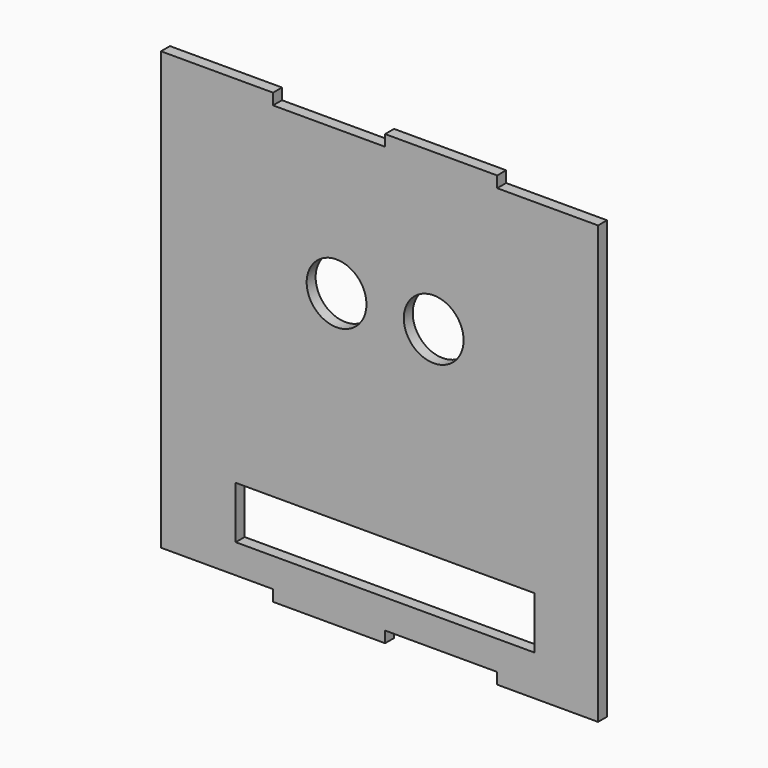
from build123d import *

# Parameters (mm, degrees)
F0_W     = 80
F0_H     = 14
F0_R     = 8
F1_DEPTH = 1.5


# Not quite as in the source:
# - a feature names something its author has since deleted; it is built from what else it names


with BuildPart() as f1:
    # F0 (on Front) → F1 (new body, symmetric)
    with BuildSketch(Plane.XZ):
        Polygon((-30, -2.9994321861), (0, -2.9994321861), (0, 0), (30, 0), (30, -2.9994321861), (57, -2.9994321861), (57, 114.0005678139), (30, 114.0005678139), (30, 117.0005678139), (0, 117.0005678139), (0, 114.0005678139), (-30, 114.0005678139), (-30, 117.0005678139), (-60, 117.0005678139), (-60, 0), (-30, 0), align=None)
        with Locations((0, 14.8116284981)):
            Rectangle(F0_W, F0_H, mode=Mode.SUBTRACT)
        with Locations((-13, 75.2281695604)):
            Circle(F0_R, mode=Mode.SUBTRACT)
        with Locations((13, 75.2218647463)):
            Circle(F0_R, mode=Mode.SUBTRACT)
    extrude(amount=F1_DEPTH, both=True)


solid = f1.part
